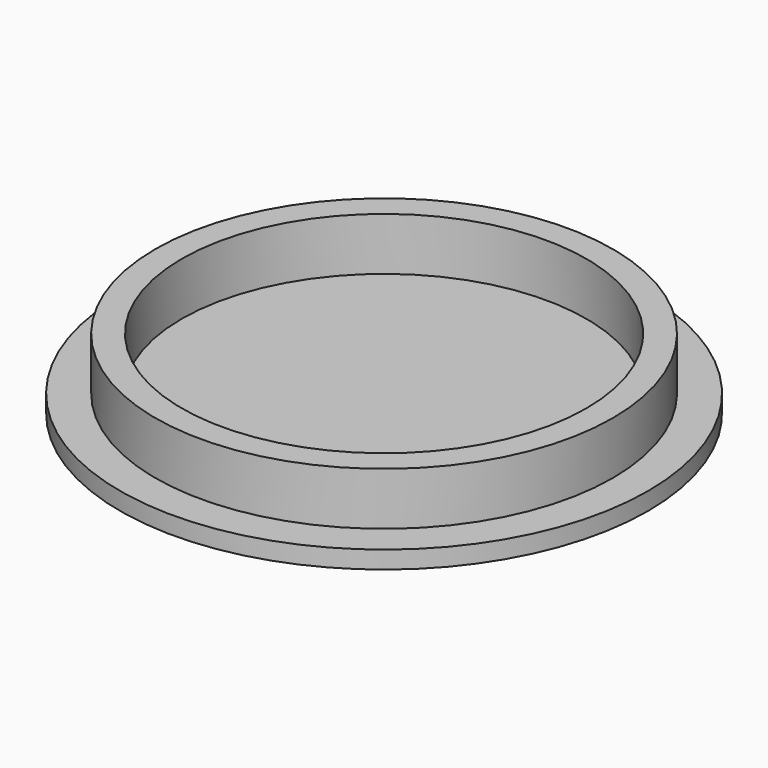
from build123d import *

# Parameters (mm, degrees)
F0_R     = 30
F1_DEPTH = 2
F2_W     = 3
F2_H     = 8


# Not quite as in the source:
# - the program builds the solid bodies; features that only make, move or delete a surface that nothing else refers to are left out


with BuildPart() as f1:
    # F0 (on Top) → F1 (new body)
    with BuildSketch(Plane.XY):
        Circle(F0_R)
    extrude(amount=F1_DEPTH)

    # F2 (on Front) → F3 (revolve)
    with BuildSketch(Plane.XZ):
        with Locations((24.5, 4)):
            Rectangle(F2_W, F2_H)
    revolve(axis=Axis((0, 0, 15.4871546511), (0, 0, 1)))


solid = f1.part
